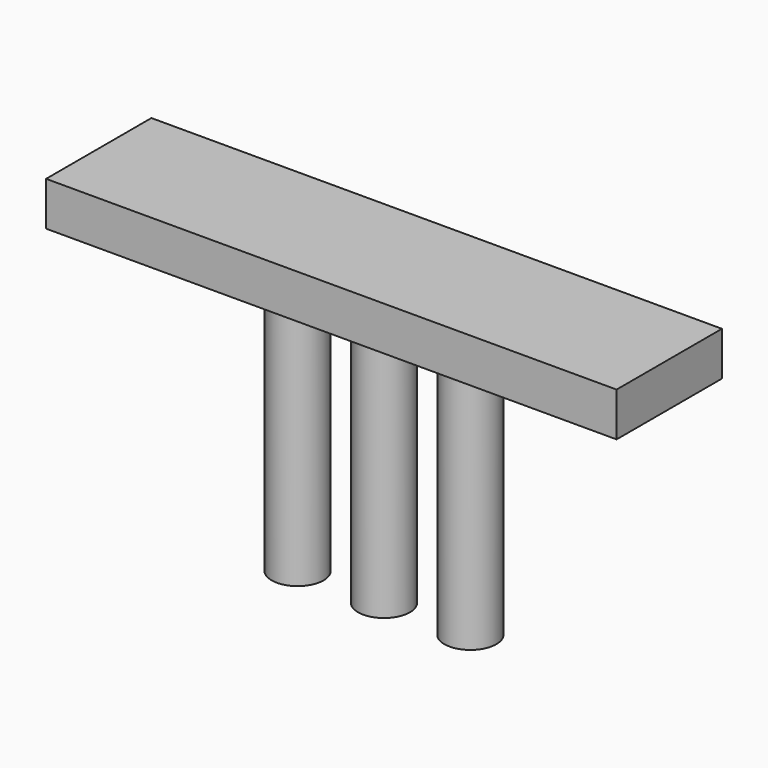
from build123d import *

# Parameters (mm, degrees)
F0_W     = 165.1
F0_H     = 38.1
F0_R     = 7.5
F1_DEPTH = 12.7
F2_DEPTH = 76.2


with BuildPart() as f1:
    # F0 (on Top) → F1 (new body)
    with BuildSketch(Plane.XY):
        Rectangle(F0_W, F0_H)
        with Locations((-25, 0)):
            Circle(F0_R, mode=Mode.SUBTRACT)
        with BuildLine():
            ThreePointArc((-7.5, 0), (0, 7.5), (7.5, 0))
            ThreePointArc((7.5, 0), (0, -7.5), (-7.5, 0))
        make_face(mode=Mode.SUBTRACT)
        with BuildLine():
            ThreePointArc((32.5, 0), (25, -7.5), (17.5, 0))
            ThreePointArc((17.5, 0), (25, 7.5), (32.5, 0))
        make_face(mode=Mode.SUBTRACT)
        with BuildLine():
            ThreePointArc((-7.5, 0), (0, -7.5), (7.5, 0))
            ThreePointArc((7.5, 0), (0, 7.5), (-7.5, 0))
        make_face()
        with Locations((-25, 0)):
            Circle(F0_R)
        with BuildLine():
            ThreePointArc((32.5, 0), (25, 7.5), (17.5, 0))
            ThreePointArc((17.5, 0), (25, -7.5), (32.5, 0))
        make_face()
    extrude(amount=F1_DEPTH)


with BuildPart() as f2:
    # F0 (on Top) → F2 (new body)
    with BuildSketch(Plane.XY):
        with BuildLine():
            ThreePointArc((-7.5, 0), (0, -7.5), (7.5, 0))
            ThreePointArc((7.5, 0), (0, 7.5), (-7.5, 0))
        make_face()
    extrude(amount=-F2_DEPTH)


with BuildPart() as f2b:
    # F0 (on Top) → F2, piece 2 (new body)
    with BuildSketch(Plane.XY):
        with Locations((-25, 0)):
            Circle(F0_R)
    extrude(amount=-F2_DEPTH)


with BuildPart() as f2c:
    # F0 (on Top) → F2, piece 3 (new body)
    with BuildSketch(Plane.XY):
        with BuildLine():
            ThreePointArc((32.5, 0), (25, 7.5), (17.5, 0))
            ThreePointArc((17.5, 0), (25, -7.5), (32.5, 0))
        make_face()
    extrude(amount=-F2_DEPTH)


solid = Compound([f1.part, f2.part, f2b.part, f2c.part])
